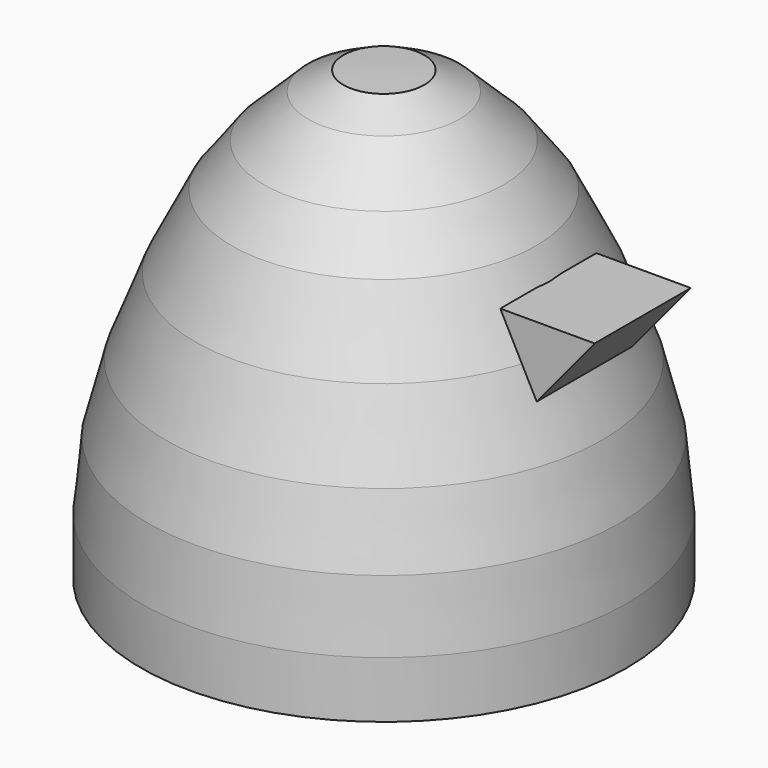
from build123d import *

# Parameters (mm, degrees)
F3_DEPTH = 12.7


# Not quite as in the source:
# - the program builds the solid bodies; features that only make, move or delete a surface that nothing else refers to are left out


with BuildPart() as f1:
    # F0 (on Front) → F1 (revolve)
    with BuildSketch(Plane.XZ):
        Polygon((8.5572190583, 45.7811206579), (0, 46.0663624108), (0, -48.9187687635), (51.3433143497, -48.9187687635), (51.3433143497, -36.9386635721), (49.9171130359, -22.3913900554), (46.2089851499, -8.1293582916), (39.9336926639, 8.1293582916), (32.2321914136, 23.5323533416), (25.386415422, 32.6600521803), (15.973476693, 41.7877547443), align=None)
    revolve(axis=Axis((0, 0, -1.4262031764), (0, 0, -1)))


with BuildPart() as f3:
    # F2 (on Front) → F3 (new body, symmetric)
    with BuildSketch(Plane.XZ):
        Polygon((54.7662004828, 17.8275406361), (34.7993597388, 17.8275406361), (42.5008572638, 2.9950267635), align=None)
    extrude(amount=F3_DEPTH, both=True)


with BuildPart() as f3_1:
    # F5: moved
    add(f3.part)


solid = Compound([f1.part, f3_1.part])
